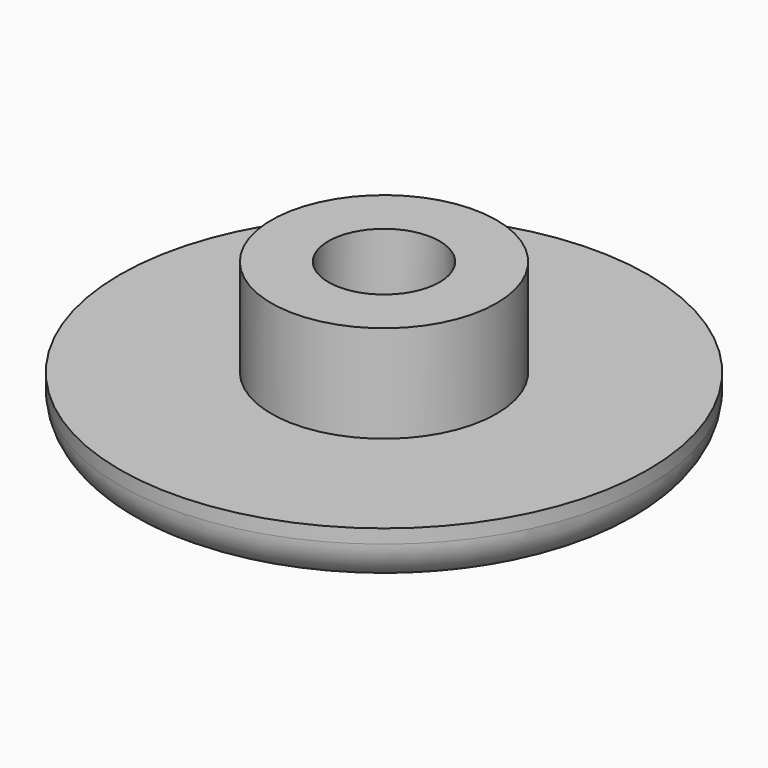
from build123d import *

# Parameters (mm, degrees)
F0_R     = 9.5
F0_R_2   = 4.05
F0_R_3   = 2
F1_DEPTH = 2
F2_R     = 4.05
F2_R_2   = 2
F3_DEPTH = 5.5
F4_R     = 1.5


# Not quite as in the source:
# - a feature names something its author has since deleted; it is built from what else it names


with BuildPart() as f1:
    # F0 (on Top) → F1 (new body)
    with BuildSketch(Plane.XY):
        Circle(F0_R)
        Circle(F0_R_2, mode=Mode.SUBTRACT)
        Circle(F0_R_2)
        Circle(F0_R_3, mode=Mode.SUBTRACT)
        Circle(F0_R_3)
    extrude(amount=F1_DEPTH)

    # F2 (on Top) → F3 (join)
    with BuildSketch(Plane.XY):
        Circle(F2_R)
        Circle(F2_R_2, mode=Mode.SUBTRACT)
    extrude(amount=F3_DEPTH)

    # F4
    f4_edges = [f1.edges().sort_by_distance(p)[0] for p in [
        (-9.5, 0, 0),
    ]]
    fillet(f4_edges, radius=F4_R)

    # F5 (on Front) → F6 (revolve, cut)
    with BuildSketch(Plane.XZ):
        with BuildLine():
            ThreePointArc((0, 0), (23.1570723538, -9.489364109), (32.9962119038, -32.5))
            ThreePointArc((32.9962119038, -32.5), (23.510635891, -8.8429276462), (0, 1))
            Line((0, 1), (0, 0))
        make_face()
    revolve(axis=Axis((0, 0, -31.5146126637), (0, 0, -1)), mode=Mode.SUBTRACT)


solid = f1.part
